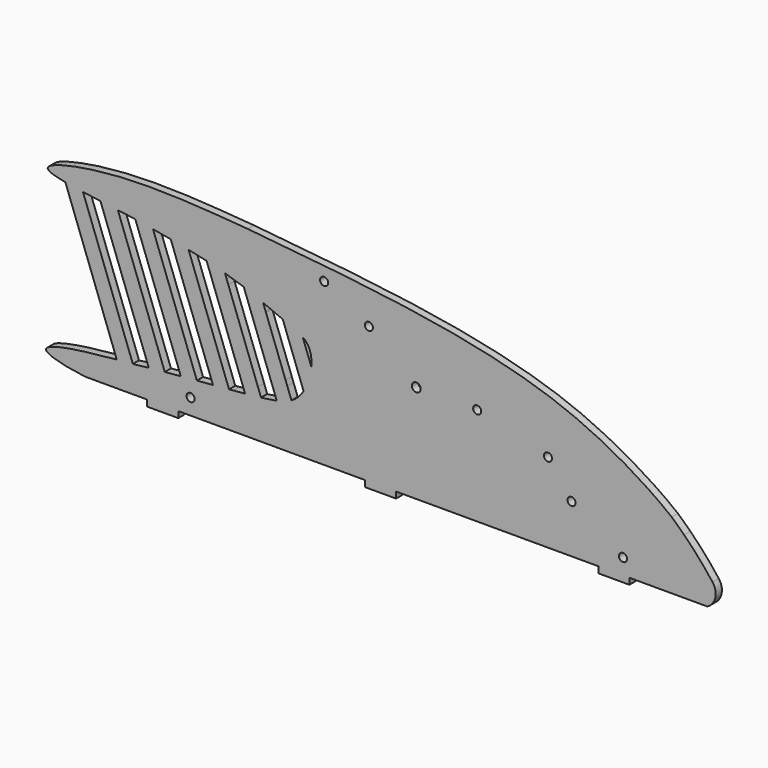
from build123d import *

# Parameters (mm, degrees)
F0_R     = 1.651
F0_R_2   = 1.8061142709
F1_DEPTH = 3.175


# Not quite as in the source:
# - a feature names something its author has since deleted; it is built from what else it names


with BuildPart() as f1:
    # F0 (on Front) → F1 (new body)
    with BuildSketch(Plane.XZ):
        with BuildLine():
            ThreePointArc((101.8242157669, -34.1397491809), (105.0796274749, -29.8955539863), (103.9375609563, -24.6699839404))
            ThreePointArc((103.9375609563, -24.6699839404), (98.381388832, -17.8735015058), (92.3581534987, -11.4872774041))
            ThreePointArc((92.3581534987, -11.4872774041), (89.8156936987, -9.0464347562), (87.2048720291, -6.6788569061))
            add(Edge.make_bspline(
                [(-85.6485664845, 40.5249372125), (-39.2165341594, 36.1134948801), (36.8475640649, 28.8975243931), (80.1105527935, -0.9081621475), (87.2048720291, -6.6788569061)],
                knots=[0, 0, 0, 0, 0.5343700027, 0.8750592741, 0.8750592741, 0.8750592741, 0.8750592741], degree=3))
            add(Edge.make_bspline(
                [(-166.859932426, 35.0105393748), (-167.0070818966, 35.1094314632), (-169.6480449533, 37.3313494106), (-138.9852615834, 44.7442194884), (-106.1222539211, 42.1445401212), (-85.6485664845, 40.5249372125)],
                knots=[0.4925129556, 0.4925129556, 0.4925129556, 0.4925129556, 0.5013804687, 0.6893595213, 1, 1, 1, 1], degree=3))
            add(Edge.make_bspline(
                [(-146.0141042884, 31.2589722541), (-151.9382775254, 32.1444047313), (-162.145842511, 33.6407441013), (-165.5296880535, 34.4446355916), (-166.859932426, 35.0105393748)],
                knots=[0.8656758918, 0.8656758918, 0.8656758918, 0.8656758918, 0.9278141873, 0.9914511144, 0.9914511144, 0.9914511144, 0.9914511144], degree=3))
            add(Edge.make_bspline(
                [(-133.5820238569, 29.35678448), (-137.9542479512, 30.0482442774), (-142.1697190197, 30.6843868334), (-146.0141042884, 31.2589722541)],
                knots=[0.8253523668, 0.8253523668, 0.8253523668, 0.8253523668, 0.8656758918, 0.8656758918, 0.8656758918, 0.8656758918], degree=3))
            add(Edge.make_bspline(
                [(-131.6806362519, 29.0942226068), (-132.3147563317, 29.1827732819), (-132.9488163176, 29.2702687124), (-133.5820238569, 29.35678448)],
                knots=[0.30311068, 0.30311068, 0.30311068, 0.30311068, 0.3105996727, 0.3105996727, 0.3105996727, 0.3105996727], degree=3))
            add(Edge.make_bspline(
                [(-124.5242243366, 28.0398482977), (-126.8819557506, 28.4091365836), (-129.2817260182, 28.759230659), (-131.6806362519, 29.0942226068)],
                knots=[0.2747794194, 0.2747794194, 0.2747794194, 0.2747794194, 0.30311068, 0.30311068, 0.30311068, 0.30311068], degree=3))
            add(Edge.make_bspline(
                [(-108.0116674089, 24.7705738209), (-112.7672708675, 26.0305747461), (-118.5089286797, 27.097680666), (-124.5242243366, 28.0398482977)],
                knots=[0.2024976878, 0.2024976878, 0.2024976878, 0.2024976878, 0.2747794194, 0.2747794194, 0.2747794194, 0.2747794194], degree=3))
            add(Edge.make_bspline(
                [(-102.5692031738, 23.558947235), (-104.3187177416, 23.9711384495), (-106.1393069255, 24.3752013047), (-108.0116674089, 24.7705738209)],
                knots=[0.7293104708, 0.7293104708, 0.7293104708, 0.7293104708, 0.7473852474, 0.7473852474, 0.7473852474, 0.7473852474], degree=3))
            add(Edge.make_bspline(
                [(-95.0830440369, 21.6100757598), (-96.2557735003, 21.9486690604), (-98.6537948613, 22.6077844658), (-101.252827931, 23.2488050276), (-102.5692031738, 23.558947235)],
                knots=[0.7016123961, 0.7016123961, 0.7016123961, 0.7016123961, 0.7157105906, 0.7293104708, 0.7293104708, 0.7293104708, 0.7293104708], degree=3))
            add(Edge.make_bspline(
                [(-87.404438233, 19.139158951), (-89.7270643692, 19.9661134917), (-92.2671026681, 20.7970503245), (-95.0830440369, 21.6100757598)],
                knots=[0.6677600115, 0.6677600115, 0.6677600115, 0.6677600115, 0.7016123961, 0.7016123961, 0.7016123961, 0.7016123961], degree=3))
            add(Edge.make_bspline(
                [(-79.5009681977, 16.0582584803), (-81.8655489773, 17.0490997411), (-84.4603298418, 18.0909300672), (-87.404438233, 19.139158951)],
                knots=[0.6248494938, 0.6248494938, 0.6248494938, 0.6248494938, 0.6677600115, 0.6677600115, 0.6677600115, 0.6677600115], degree=3))
            add(Edge.make_bspline(
                [(-71.4843313159, 12.6703730925), (-73.9521121546, 13.6621239816), (-76.5468977698, 14.8204006358), (-79.5009681977, 16.0582584803)],
                knots=[0.5712413903, 0.5712413903, 0.5712413903, 0.5712413903, 0.6248494938, 0.6248494938, 0.6248494938, 0.6248494938], degree=3))
            add(Edge.make_bspline(
                [(-63.3356655994, 8.9243363369), (-65.4352611539, 10.424736107), (-68.3578707481, 11.4139122272), (-71.4843313159, 12.6703730925)],
                knots=[0.5033246535, 0.5033246535, 0.5033246535, 0.5033246535, 0.5712413903, 0.5712413903, 0.5712413903, 0.5712413903], degree=3))
            add(Edge.make_bspline(
                [(-59.8424153153, -0.5517176671), (-59.5685681737, 2.4835120245), (-60.1606540756, 6.1658647467), (-62.6477224268, 8.4327227136), (-63.3356655994, 8.9243363369)],
                knots=[0.4110186684, 0.4110186684, 0.4110186684, 0.4110186684, 0.4810713889, 0.5033246535, 0.5033246535, 0.5033246535, 0.5033246535], degree=3))
            add(Edge.make_bspline(
                [(-63.0075179076, -10.3244698493), (-61.5384136321, -7.9164198493), (-60.3388409827, -4.449568462), (-59.8949280547, -1.1337512231), (-59.8424153153, -0.5517176671)],
                knots=[0.3356359982, 0.3356359982, 0.3356359982, 0.3356359982, 0.3975854069, 0.4110186684, 0.4110186684, 0.4110186684, 0.4110186684], degree=3))
            add(Edge.make_bspline(
                [(-67.9444449918, -15.2908373738), (-67.2102943656, -14.8703950623), (-65.3380336592, -13.5477151393), (-63.8223020979, -11.6600054557), (-63.0075179076, -10.3244698493)],
                knots=[0.2815826078, 0.2815826078, 0.2815826078, 0.2815826078, 0.3012780567, 0.3356359982, 0.3356359982, 0.3356359982, 0.3356359982], degree=3))
            add(Edge.make_bspline(
                [(-73.9382749374, -17.3901705387), (-71.6234415545, -16.908346885), (-69.6446238077, -16.2645164604), (-67.9444449918, -15.2908373738)],
                knots=[0.2359710075, 0.2359710075, 0.2359710075, 0.2359710075, 0.2815826078, 0.2815826078, 0.2815826078, 0.2815826078], degree=3))
            add(Edge.make_bspline(
                [(-80.3548864441, -18.3426345759), (-77.9680739947, -18.0724427195), (-75.8398049281, -17.785966683), (-73.9382749374, -17.3901705387)],
                knots=[0.1985031592, 0.1985031592, 0.1985031592, 0.1985031592, 0.2359710075, 0.2359710075, 0.2359710075, 0.2359710075], degree=3))
            add(Edge.make_bspline(
                [(-81.2421848416, -18.4411984354), (-80.9425135443, -18.4084739112), (-80.6467668076, -18.3756760061), (-80.3548864685, -18.3426345786)],
                knots=[0.1939212624, 0.1939212624, 0.1939212624, 0.1939212624, 0.1985031592, 0.1985031592, 0.1985031592, 0.1985031592], degree=3))
            add(Edge.make_bspline(
                [(-81.242184815, -18.4411984325), (-86.8235115185, -20.9425074888), (-91.5502384252, -21.2149262437), (-96.0113873436, -21.2686423497)],
                knots=[0.706684877, 0.706684877, 0.706684877, 0.706684877, 0.9497553414, 0.9497553414, 0.9497553414, 0.9497553414], degree=3))
            add(Edge.make_bspline(
                [(-96.0113873436, -21.2686423497), (-96.9335434145, -21.2797459094), (-97.8443517945, -21.2815046809), (-98.7490148928, -21.2916732166)],
                knots=[0.9497553414, 0.9497553414, 0.9497553414, 0.9497553414, 1, 1, 1, 1], degree=3))
            add(Edge.make_bspline(
                [(-133.305364874, -23.3117086185), (-122.8338263442, -22.475714872), (-110.8834436824, -21.7895004957), (-98.7490148928, -21.2916732166)],
                knots=[0.853722198, 0.853722198, 0.853722198, 0.853722198, 0.9841655102, 0.9841655102, 0.9841655102, 0.9841655102], degree=3))
            add(Edge.make_bspline(
                [(-139.2463766665, -23.8169718217), (-137.328523595, -23.6430585147), (-135.3449969617, -23.4745423478), (-133.305364874, -23.3117086185)],
                knots=[0.8283146263, 0.8283146263, 0.8283146263, 0.8283146263, 0.853722198, 0.853722198, 0.853722198, 0.853722198], degree=3))
            add(Edge.make_bspline(
                [(-152.2580874144, -34.1547166765), (-161.5981584725, -33.009893689), (-177.1137531043, -28.7902056183), (-155.6923384135, -25.3083121314), (-139.2463766665, -23.8169718217)],
                knots=[0.4265501578, 0.4265501578, 0.4265501578, 0.4265501578, 0.610439776, 0.8283146263, 0.8283146263, 0.8283146263, 0.8283146263], degree=3))
            ThreePointArc((-152.2580874144, -34.1547166765), (-152.2495450174, -34.155500254), (-152.2409707448, -34.1557617705))
            Line((-152.2409707448, -34.1557617705), (-126.8495585793, -34.1557617705))
            Line((-126.8495585793, -34.1557617705), (-126.8495585793, -35.5765540648))
            add(Edge.make_bspline(
                [(-114.1495585793, -35.5765321102), (-118.523301185, -35.6218647567), (-122.7687076518, -35.6265709825), (-126.8495585793, -35.5765540648)],
                knots=[0.2221019343, 0.2221019343, 0.2221019343, 0.2221019343, 0.2834552379, 0.2834552379, 0.2834552379, 0.2834552379], degree=3))
            Line((-114.1495585793, -35.5765321102), (-114.1495585793, -34.1557617705))
            Line((-114.1495585793, -34.1557617705), (-63.3228805236, -34.1557617705))
            Line((-63.3228805236, -34.1557617705), (-57.4806444347, -34.1557617705))
            Line((-57.4806444347, -34.1557617705), (-37.9495585793, -34.1557617705))
            Line((-37.9495585793, -34.1557617705), (-37.9495585793, -36.6983525455))
            Line((-37.9495585793, -36.6983525455), (-25.2495585793, -36.6983525455))
            Line((-25.2495585793, -36.6983525455), (-25.2495585793, -34.1583525455))
            Line((-25.2495585793, -34.1583525455), (-25.2495585793, -34.1557617705))
            Line((-25.2495585793, -34.1557617705), (57.3004414207, -34.1557617705))
            Line((57.3004414207, -34.1557617705), (57.3004414207, -36.6957617705))
            Line((57.3004414207, -36.6957617705), (70.0004414207, -36.6957617705))
            Line((70.0004414207, -36.6957617705), (70.0004414207, -34.1557617705))
            Line((70.0004414207, -34.1557617705), (101.7590292552, -34.1557617705))
            ThreePointArc((101.7590292552, -34.1557617705), (101.7925914524, -34.1516999913), (101.8242157669, -34.1397491809))
        make_face()
        with Locations((-109.1138124466, -27.6470873505)):
            Circle(F0_R, mode=Mode.SUBTRACT)
        with Locations((67.3906803131, -27.7224443853)):
            Circle(F0_R, mode=Mode.SUBTRACT)
        with Locations((46.3759977302, -14.4284265014)):
            Circle(F0_R, mode=Mode.SUBTRACT)
        with Locations((36.7670959526, -1.6008562954)):
            Circle(F0_R, mode=Mode.SUBTRACT)
        with Locations((-36.3425172139, 21.5731277197)):
            Circle(F0_R, mode=Mode.SUBTRACT)
        with Locations((-54.6054057777, 31.7963883281)):
            Circle(F0_R, mode=Mode.SUBTRACT)
        with Locations((-17.0012986666, 5.9441462856)):
            Circle(F0_R_2, mode=Mode.SUBTRACT)
        with Locations((7.8653013334, 5.9441462856)):
            Circle(F0_R, mode=Mode.SUBTRACT)
        with BuildLine():
            add(Edge.make_bspline(
                [(-146.0141042884, 31.2589722541), (-151.9382775254, 32.1444047313), (-162.145842511, 33.6407441013), (-165.5296880535, 34.4446355916), (-166.859932426, 35.0105393748)],
                knots=[0.8656758918, 0.8656758918, 0.8656758918, 0.8656758918, 0.9278141873, 0.9914511144, 0.9914511144, 0.9914511144, 0.9914511144], degree=3))
            add(Edge.make_bspline(
                [(-160.2262755413, 33.0946831043), (-163.4901021945, 33.703641199), (-165.8451335745, 34.3285418292), (-166.859932426, 35.0105393748)],
                knots=[0.4313592041, 0.4313592041, 0.4313592041, 0.4313592041, 0.4925129556, 0.4925129556, 0.4925129556, 0.4925129556], degree=3))
            add(Edge.make_bspline(
                [(-153.0349213305, 31.9455216907), (-155.7238859248, 32.329156746), (-158.1576206982, 32.7087177189), (-160.2262755413, 33.0946831043)],
                knots=[0.3925991786, 0.3925991786, 0.3925991786, 0.3925991786, 0.4313592041, 0.4313592041, 0.4313592041, 0.4313592041], degree=3))
            add(Edge.make_bspline(
                [(-145.911513117, 30.9806757105), (-148.4188378285, 31.3090067169), (-150.8139400572, 31.6286538986), (-153.0349213305, 31.9455216907)],
                knots=[0.3605848892, 0.3605848892, 0.3605848892, 0.3605848892, 0.3925991786, 0.3925991786, 0.3925991786, 0.3925991786], degree=3))
            Line((-145.911513117, 30.9806757105), (-146.0141042884, 31.2589722541))
        make_face()
        with BuildLine():
            add(Edge.make_bspline(
                [(-133.5820238569, 29.35678448), (-137.9542479512, 30.0482442774), (-142.1697190197, 30.6843868334), (-146.0141042884, 31.2589722541)],
                knots=[0.8253523668, 0.8253523668, 0.8253523668, 0.8253523668, 0.8656758918, 0.8656758918, 0.8656758918, 0.8656758918], degree=3))
            Line((-146.0141042884, 31.2589722541), (-145.911513117, 30.9806757105))
            add(Edge.make_bspline(
                [(-138.8022091808, 30.0540900559), (-141.2342218587, 30.373212682), (-143.6197455711, 30.6805716428), (-145.911513117, 30.9806757105)],
                knots=[0.3313228996, 0.3313228996, 0.3313228996, 0.3313228996, 0.3605848892, 0.3605848892, 0.3605848892, 0.3605848892], degree=3))
            add(Edge.make_bspline(
                [(-133.5820238569, 29.35678448), (-135.3342092326, 29.5961872878), (-137.0798672845, 29.8280886563), (-138.8022091808, 30.0540900559)],
                knots=[0.3105996727, 0.3105996727, 0.3105996727, 0.3105996727, 0.3313228996, 0.3313228996, 0.3313228996, 0.3313228996], degree=3))
        make_face()
        with BuildLine():
            add(Edge.make_bspline(
                [(-153.0349213305, 31.9455216907), (-155.7238859248, 32.329156746), (-158.1576206982, 32.7087177189), (-160.2262755413, 33.0946831043)],
                knots=[0.3925991786, 0.3925991786, 0.3925991786, 0.3925991786, 0.4313592041, 0.4313592041, 0.4313592041, 0.4313592041], degree=3))
            Line((-160.2262755413, 33.0946831043), (-139.2463766665, -23.8169718217))
            add(Edge.make_bspline(
                [(-139.2463766665, -23.8169718217), (-137.328523595, -23.6430585147), (-135.3449969617, -23.4745423478), (-133.305364874, -23.3117086185)],
                knots=[0.8283146263, 0.8283146263, 0.8283146263, 0.8283146263, 0.853722198, 0.853722198, 0.853722198, 0.853722198], degree=3))
            add(Edge.make_bspline(
                [(-133.305364874, -23.3117086185), (-133.1004170164, -23.2884499459), (-132.895464166, -23.2652975185), (-132.6905143301, -23.2422500801)],
                knots=[0, 0, 0, 0, 0.0020208288, 0.0020208288, 0.0020208288, 0.0020208288], degree=3))
            Line((-132.6905143301, -23.2422500801), (-153.0349213305, 31.9455216907))
        make_face()
        with BuildLine():
            add(Edge.make_bspline(
                [(-131.6806362519, 29.0942226068), (-132.3147563317, 29.1827732819), (-132.9488163176, 29.2702687124), (-133.5820238569, 29.35678448)],
                knots=[0.30311068, 0.30311068, 0.30311068, 0.30311068, 0.3105996727, 0.3105996727, 0.3105996727, 0.3105996727], degree=3))
            add(Edge.make_bspline(
                [(-131.6649143971, 29.0515743188), (-132.3068274232, 29.1544685142), (-132.9460837508, 29.2562116349), (-133.5820238569, 29.35678448)],
                knots=[0.8194873091, 0.8194873091, 0.8194873091, 0.8194873091, 0.8253523668, 0.8253523668, 0.8253523668, 0.8253523668], degree=3))
            Line((-131.6649143971, 29.0515743188), (-131.6806362519, 29.0942226068))
        make_face()
        with BuildLine():
            add(Edge.make_bspline(
                [(-138.8022091808, 30.0540900559), (-141.2342218587, 30.373212682), (-143.6197455711, 30.6805716428), (-145.911513117, 30.9806757105)],
                knots=[0.3313228996, 0.3313228996, 0.3313228996, 0.3313228996, 0.3605848892, 0.3605848892, 0.3605848892, 0.3605848892], degree=3))
            Line((-145.911513117, 30.9806757105), (-126.2084949262, -22.4672164347))
            Line((-126.2084949262, -22.4672164347), (-126.1805877741, -22.5429194788))
            add(Edge.make_bspline(
                [(-126.1805877741, -22.5429194788), (-123.9904993464, -22.3178624533), (-121.8105472714, -22.1033724676), (-119.6506417586, -21.8978951719)],
                knots=[0.0234517677, 0.0234517677, 0.0234517677, 0.0234517677, 0.0451483955, 0.0451483955, 0.0451483955, 0.0451483955], degree=3))
            Line((-119.6506417586, -21.8978951719), (-138.8022091808, 30.0540900559))
        make_face()
        with BuildLine():
            Line((-131.6806362519, 29.0942226068), (-131.6649143971, 29.0515743188))
            add(Edge.make_bspline(
                [(-124.4587574049, 27.8622577646), (-126.8749129775, 28.2738277576), (-129.2881250019, 28.6705915024), (-131.6649143971, 29.0515743188)],
                knots=[0.7977709605, 0.7977709605, 0.7977709605, 0.7977709605, 0.8194873091, 0.8194873091, 0.8194873091, 0.8194873091], degree=3))
            Line((-124.4587574049, 27.8622577646), (-124.5242243366, 28.0398482977))
            add(Edge.make_bspline(
                [(-124.5242243366, 28.0398482977), (-126.8819557506, 28.4091365836), (-129.2817260182, 28.759230659), (-131.6806362519, 29.0942226068)],
                knots=[0.2747794194, 0.2747794194, 0.2747794194, 0.2747794194, 0.30311068, 0.30311068, 0.30311068, 0.30311068], degree=3))
        make_face()
        with BuildLine():
            add(Edge.make_bspline(
                [(-124.4587574049, 27.8622577646), (-126.8749129775, 28.2738277576), (-129.2881250019, 28.6705915024), (-131.6649143971, 29.0515743188)],
                knots=[0.7977709605, 0.7977709605, 0.7977709605, 0.7977709605, 0.8194873091, 0.8194873091, 0.8194873091, 0.8194873091], degree=3))
            Line((-131.6649143971, 29.0515743188), (-113.1052410481, -21.2947944356))
            add(Edge.make_bspline(
                [(-113.1052410481, -21.2947944356), (-110.8824432445, -21.0958896664), (-108.6931707163, -20.9052358248), (-106.5490323993, -20.7210121272)],
                knots=[0.0673104273, 0.0673104273, 0.0673104273, 0.0673104273, 0.0901819686, 0.0901819686, 0.0901819686, 0.0901819686], degree=3))
            Line((-106.5490323993, -20.7210121272), (-124.4587574049, 27.8622577646))
        make_face()
        with BuildLine():
            add(Edge.make_bspline(
                [(-132.6905143301, -23.2422500801), (-130.5170162436, -22.9978314259), (-128.3438571985, -22.7652205402), (-126.1805877741, -22.5429194788)],
                knots=[0.0020208288, 0.0020208288, 0.0020208288, 0.0020208288, 0.0234517677, 0.0234517677, 0.0234517677, 0.0234517677], degree=3))
            add(Edge.make_bspline(
                [(-133.305364874, -23.3117086185), (-133.1004170164, -23.2884499459), (-132.895464166, -23.2652975185), (-132.6905143301, -23.2422500801)],
                knots=[0, 0, 0, 0, 0.0020208288, 0.0020208288, 0.0020208288, 0.0020208288], degree=3))
            add(Edge.make_bspline(
                [(-133.305364874, -23.3117086185), (-122.8338263442, -22.475714872), (-110.8834436824, -21.7895004957), (-98.7490148928, -21.2916732166)],
                knots=[0.853722198, 0.853722198, 0.853722198, 0.853722198, 0.9841655102, 0.9841655102, 0.9841655102, 0.9841655102], degree=3))
            add(Edge.make_bspline(
                [(-98.7490148928, -21.2916732166), (-97.7639622967, -21.2512604323), (-96.7776968514, -21.2120891039), (-95.7909112202, -21.174179885)],
                knots=[0.9841655102, 0.9841655102, 0.9841655102, 0.9841655102, 0.9947546797, 0.9947546797, 0.9947546797, 0.9947546797], degree=3))
            add(Edge.make_bspline(
                [(-91.8007028901, -19.4584197408), (-93.1232258666, -20.0303526691), (-94.4561565841, -20.6022678336), (-95.7909112202, -21.174179885)],
                knots=[0.9537015671, 0.9537015671, 0.9537015671, 0.9537015671, 0.9918863691, 0.9918863691, 0.9918863691, 0.9918863691], degree=3))
            add(Edge.make_bspline(
                [(-93.4265039677, -19.6008757346), (-92.8786151945, -19.5531958217), (-92.336588061, -19.5057251461), (-91.8007028901, -19.4584197408)],
                knots=[0.1394929365, 0.1394929365, 0.1394929365, 0.1394929365, 0.1461036875, 0.1461036875, 0.1461036875, 0.1461036875], degree=3))
            add(Edge.make_bspline(
                [(-99.987241926, -20.1623714966), (-97.7243605002, -19.9704519625), (-95.5321437404, -19.784118622), (-93.4265039677, -19.6008757346)],
                knots=[0.1140865752, 0.1140865752, 0.1140865752, 0.1140865752, 0.1394929365, 0.1394929365, 0.1394929365, 0.1394929365], degree=3))
            add(Edge.make_bspline(
                [(-106.5490323993, -20.7210121272), (-104.3080473179, -20.5284673856), (-102.1163657866, -20.342946782), (-99.987241926, -20.1623714966)],
                knots=[0.0901819686, 0.0901819686, 0.0901819686, 0.0901819686, 0.1140865752, 0.1140865752, 0.1140865752, 0.1140865752], degree=3))
            add(Edge.make_bspline(
                [(-113.1052410481, -21.2947944356), (-110.8824432445, -21.0958896664), (-108.6931707163, -20.9052358248), (-106.5490323993, -20.7210121272)],
                knots=[0.0673104273, 0.0673104273, 0.0673104273, 0.0673104273, 0.0901819686, 0.0901819686, 0.0901819686, 0.0901819686], degree=3))
            add(Edge.make_bspline(
                [(-119.6506417586, -21.8978951719), (-117.4444051423, -21.6880102808), (-115.2590843306, -21.4875288805), (-113.1052410481, -21.2947944356)],
                knots=[0.0451483955, 0.0451483955, 0.0451483955, 0.0451483955, 0.0673104273, 0.0673104273, 0.0673104273, 0.0673104273], degree=3))
            add(Edge.make_bspline(
                [(-126.1805877741, -22.5429194788), (-123.9904993464, -22.3178624533), (-121.8105472714, -22.1033724676), (-119.6506417586, -21.8978951719)],
                knots=[0.0234517677, 0.0234517677, 0.0234517677, 0.0234517677, 0.0451483955, 0.0451483955, 0.0451483955, 0.0451483955], degree=3))
        make_face()
        with BuildLine():
            Line((-124.5242243366, 28.0398482977), (-124.4587574049, 27.8622577646))
            add(Edge.make_bspline(
                [(-117.2187514903, 26.5811200726), (-119.6125726628, 27.0223849911), (-122.0371434652, 27.4497579888), (-124.4587574049, 27.8622577646)],
                knots=[0.7760055522, 0.7760055522, 0.7760055522, 0.7760055522, 0.7977709605, 0.7977709605, 0.7977709605, 0.7977709605], degree=3))
            add(Edge.make_bspline(
                [(-109.9305159939, 25.1691511818), (-112.3022395164, 25.6539310572), (-114.7440643866, 26.1249487363), (-117.2187514903, 26.5811200726)],
                knots=[0.7535048843, 0.7535048843, 0.7535048843, 0.7535048843, 0.7760055522, 0.7760055522, 0.7760055522, 0.7760055522], degree=3))
            add(Edge.make_bspline(
                [(-108.0116674089, 24.7705738209), (-108.6455986912, 24.9044364015), (-109.2854646151, 25.0373027922), (-109.9305159939, 25.1691511818)],
                knots=[0.7473852474, 0.7473852474, 0.7473852474, 0.7473852474, 0.7535048843, 0.7535048843, 0.7535048843, 0.7535048843], degree=3))
            add(Edge.make_bspline(
                [(-108.0116674089, 24.7705738209), (-112.7672708675, 26.0305747461), (-118.5089286797, 27.097680666), (-124.5242243366, 28.0398482977)],
                knots=[0.2024976878, 0.2024976878, 0.2024976878, 0.2024976878, 0.2747794194, 0.2747794194, 0.2747794194, 0.2747794194], degree=3))
        make_face()
        with BuildLine():
            add(Edge.make_bspline(
                [(-114.1495585793, -35.5765321102), (-118.523301185, -35.6218647567), (-122.7687076518, -35.6265709825), (-126.8495585793, -35.5765540648)],
                knots=[0.2221019343, 0.2221019343, 0.2221019343, 0.2221019343, 0.2834552379, 0.2834552379, 0.2834552379, 0.2834552379], degree=3))
            Line((-126.8495585793, -35.5765540648), (-126.8495585793, -36.6957617705))
            Line((-126.8495585793, -36.6957617705), (-114.1495585793, -36.6957617705))
            Line((-114.1495585793, -36.6957617705), (-114.1495585793, -35.5765321102))
        make_face()
        with BuildLine():
            add(Edge.make_bspline(
                [(-98.7490148928, -21.2916732166), (-97.7639622967, -21.2512604323), (-96.7776968514, -21.2120891039), (-95.7909112202, -21.174179885)],
                knots=[0.9841655102, 0.9841655102, 0.9841655102, 0.9841655102, 0.9947546797, 0.9947546797, 0.9947546797, 0.9947546797], degree=3))
            add(Edge.make_bspline(
                [(-96.0113873436, -21.2686423497), (-96.9335434145, -21.2797459094), (-97.8443517945, -21.2815046809), (-98.7490148928, -21.2916732166)],
                knots=[0.9497553414, 0.9497553414, 0.9497553414, 0.9497553414, 1, 1, 1, 1], degree=3))
            add(Edge.make_bspline(
                [(-95.7909112202, -21.174179885), (-95.8643982082, -21.2056673906), (-95.9378907249, -21.2371548868), (-96.0113873378, -21.268642376)],
                knots=[0.9918863691, 0.9918863691, 0.9918863691, 0.9918863691, 0.9939886926, 0.9939886926, 0.9939886926, 0.9939886926], degree=3))
        make_face()
        with BuildLine():
            add(Edge.make_bspline(
                [(-109.9305159939, 25.1691511818), (-112.3022395164, 25.6539310572), (-114.7440643866, 26.1249487363), (-117.2187514903, 26.5811200726)],
                knots=[0.7535048843, 0.7535048843, 0.7535048843, 0.7535048843, 0.7760055522, 0.7760055522, 0.7760055522, 0.7760055522], degree=3))
            Line((-117.2187514903, 26.5811200726), (-99.987241926, -20.1623714966))
            add(Edge.make_bspline(
                [(-99.987241926, -20.1623714966), (-97.7243605002, -19.9704519625), (-95.5321437404, -19.784118622), (-93.4265039677, -19.6008757346)],
                knots=[0.1140865752, 0.1140865752, 0.1140865752, 0.1140865752, 0.1394929365, 0.1394929365, 0.1394929365, 0.1394929365], degree=3))
            Line((-93.4265039677, -19.6008757346), (-109.9305159939, 25.1691511818))
        make_face()
        with BuildLine():
            add(Edge.make_bspline(
                [(-91.8007028901, -19.4584197408), (-93.1232258666, -20.0303526691), (-94.4561565841, -20.6022678336), (-95.7909112202, -21.174179885)],
                knots=[0.9537015671, 0.9537015671, 0.9537015671, 0.9537015671, 0.9918863691, 0.9918863691, 0.9918863691, 0.9918863691], degree=3))
            add(Edge.make_bspline(
                [(-95.7909112202, -21.174179885), (-95.8643982082, -21.2056673906), (-95.9378907249, -21.2371548868), (-96.0113873378, -21.268642376)],
                knots=[0.9918863691, 0.9918863691, 0.9918863691, 0.9918863691, 0.9939886926, 0.9939886926, 0.9939886926, 0.9939886926], degree=3))
            add(Edge.make_bspline(
                [(-81.242184815, -18.4411984325), (-86.8235115185, -20.9425074888), (-91.5502384252, -21.2149262437), (-96.0113873436, -21.2686423497)],
                knots=[0.706684877, 0.706684877, 0.706684877, 0.706684877, 0.9497553414, 0.9497553414, 0.9497553414, 0.9497553414], degree=3))
            add(Edge.make_bspline(
                [(-86.8765772789, -19.0100525082), (-84.8769444797, -18.8209932024), (-82.9926132911, -18.6323476668), (-81.2421848416, -18.4411984354)],
                knots=[0.1671576631, 0.1671576631, 0.1671576631, 0.1671576631, 0.1939212624, 0.1939212624, 0.1939212624, 0.1939212624], degree=3))
            add(Edge.make_bspline(
                [(-91.8007028901, -19.4584197408), (-90.0940112569, -19.3077610852), (-88.4496175808, -19.1587787681), (-86.8765772789, -19.0100525082)],
                knots=[0.1461036875, 0.1461036875, 0.1461036875, 0.1461036875, 0.1671576631, 0.1671576631, 0.1671576631, 0.1671576631], degree=3))
        make_face()
        with BuildLine():
            add(Edge.make_bspline(
                [(-95.0830440369, 21.6100757598), (-96.2557735003, 21.9486690604), (-98.6537948613, 22.6077844658), (-101.252827931, 23.2488050276), (-102.5692031738, 23.558947235)],
                knots=[0.7016123961, 0.7016123961, 0.7016123961, 0.7016123961, 0.7157105906, 0.7293104708, 0.7293104708, 0.7293104708, 0.7293104708], degree=3))
            Line((-102.5692031738, 23.558947235), (-102.3586580437, 22.9878066466))
            add(Edge.make_bspline(
                [(-100.3286994702, 22.1462184152), (-100.9667307172, 22.4336146948), (-101.6422894477, 22.7143386396), (-102.3586580437, 22.9878066466)],
                knots=[0.1569312578, 0.1569312578, 0.1569312578, 0.1569312578, 0.1706574214, 0.1706574214, 0.1706574214, 0.1706574214], degree=3))
            add(Edge.make_bspline(
                [(-100.3286994703, 22.1462184152), (-98.3419538443, 21.370808658), (-96.3670610524, 20.5954191311), (-94.4231813629, 19.820082537)],
                knots=[0.0317602035, 0.0317602035, 0.0317602035, 0.0317602035, 0.0831010058, 0.0831010058, 0.0831010058, 0.0831010058], degree=3))
            Line((-94.4231813629, 19.820082537), (-95.0830440369, 21.6100757598))
        make_face()
        with BuildLine():
            add(Edge.make_bspline(
                [(-86.8765772789, -19.0100525082), (-84.8769444797, -18.8209932024), (-82.9926132911, -18.6323476668), (-81.2421848416, -18.4411984354)],
                knots=[0.1671576631, 0.1671576631, 0.1671576631, 0.1671576631, 0.1939212624, 0.1939212624, 0.1939212624, 0.1939212624], degree=3))
            add(Edge.make_bspline(
                [(-80.4533326205, -18.075582058), (-80.7178914258, -18.2021897286), (-80.9809740433, -18.3241350704), (-81.242184815, -18.4411984325)],
                knots=[0.6953089753, 0.6953089753, 0.6953089753, 0.6953089753, 0.706684877, 0.706684877, 0.706684877, 0.706684877], degree=3))
            Line((-80.4533326205, -18.075582058), (-81.6267561876, -14.89246485))
            add(Edge.make_bspline(
                [(-81.6267561876, -14.89246485), (-83.488541827, -15.7754334505), (-85.4295143068, -16.6582668958), (-87.418121426, -17.5410190391)],
                knots=[0.8521015775, 0.8521015775, 0.8521015775, 0.8521015775, 0.9110320857, 0.9110320857, 0.9110320857, 0.9110320857], degree=3))
            Line((-87.4181214259, -17.5410190391), (-86.8765772789, -19.0100525082))
        make_face()
        with BuildLine():
            add(Edge.make_bspline(
                [(-80.4533326205, -18.075582058), (-80.7178914258, -18.2021897286), (-80.9809740433, -18.3241350704), (-81.242184815, -18.4411984325)],
                knots=[0.6953089753, 0.6953089753, 0.6953089753, 0.6953089753, 0.706684877, 0.706684877, 0.706684877, 0.706684877], degree=3))
            add(Edge.make_bspline(
                [(-81.2421848416, -18.4411984354), (-80.9425135443, -18.4084739112), (-80.6467668076, -18.3756760061), (-80.3548864685, -18.3426345786)],
                knots=[0.1939212624, 0.1939212624, 0.1939212624, 0.1939212624, 0.1985031592, 0.1985031592, 0.1985031592, 0.1985031592], degree=3))
            Line((-80.3548864441, -18.3426345759), (-80.4533326205, -18.075582058))
        make_face()
        with BuildLine():
            add(Edge.make_bspline(
                [(-100.3286994702, 22.1462184152), (-100.9667307172, 22.4336146948), (-101.6422894477, 22.7143386396), (-102.3586580437, 22.9878066466)],
                knots=[0.1569312578, 0.1569312578, 0.1569312578, 0.1569312578, 0.1706574214, 0.1706574214, 0.1706574214, 0.1706574214], degree=3))
            Line((-102.3586580437, 22.9878066466), (-102.3368731501, 22.9287113022))
            add(Edge.make_bspline(
                [(-102.3368731501, 22.9287113022), (-101.6666269569, 22.6678788806), (-100.9969926472, 22.4070475034), (-100.3286994703, 22.1462184152)],
                knots=[0.0144903994, 0.0144903994, 0.0144903994, 0.0144903994, 0.0317602035, 0.0317602035, 0.0317602035, 0.0317602035], degree=3))
        make_face()
        with BuildLine():
            add(Edge.make_bspline(
                [(-102.3368731501, 22.9287113022), (-101.6666269569, 22.6678788806), (-100.9969926472, 22.4070475034), (-100.3286994703, 22.1462184152)],
                knots=[0.0144903994, 0.0144903994, 0.0144903994, 0.0144903994, 0.0317602035, 0.0317602035, 0.0317602035, 0.0317602035], degree=3))
            Line((-102.3368731501, 22.9287113022), (-87.4181214259, -17.5410190391))
            add(Edge.make_bspline(
                [(-81.6267561876, -14.89246485), (-83.488541827, -15.7754334505), (-85.4295143068, -16.6582668958), (-87.418121426, -17.5410190391)],
                knots=[0.8521015775, 0.8521015775, 0.8521015775, 0.8521015775, 0.9110320857, 0.9110320857, 0.9110320857, 0.9110320857], degree=3))
            Line((-81.6267561876, -14.89246485), (-93.7330933839, 17.9480978737))
            add(Edge.make_bspline(
                [(-93.7330933839, 17.9480978737), (-95.3779897097, 19.4459076442), (-97.4790442928, 20.862613106), (-100.3286994702, 22.1462184152)],
                knots=[0.0956257444, 0.0956257444, 0.0956257444, 0.0956257444, 0.1569312578, 0.1569312578, 0.1569312578, 0.1569312578], degree=3))
        make_face()
        with BuildLine():
            add(Edge.make_bspline(
                [(-79.5009681977, 16.0582584803), (-81.8655489773, 17.0490997411), (-84.4603298418, 18.0909300672), (-87.404438233, 19.139158951)],
                knots=[0.6248494938, 0.6248494938, 0.6248494938, 0.6248494938, 0.6677600115, 0.6677600115, 0.6677600115, 0.6677600115], degree=3))
            Line((-87.404438233, 19.139158951), (-86.4479529651, 16.5445249237))
            add(Edge.make_bspline(
                [(-86.4479529651, 16.5445249237), (-83.569113096, 15.317450314), (-80.8356242299, 14.0906237876), (-78.3235020587, 12.8641750869)],
                knots=[0.1554096519, 0.1554096519, 0.1554096519, 0.1554096519, 0.2366858177, 0.2366858177, 0.2366858177, 0.2366858177], degree=3))
            Line((-78.3235020587, 12.8641750869), (-78.4705088009, 13.2629566556))
            Line((-78.4705088009, 13.2629566556), (-79.5009681977, 16.0582584803))
        make_face()
        with BuildLine():
            Line((-93.7330933839, 17.9480978737), (-94.4231813629, 19.820082537))
            add(Edge.make_bspline(
                [(-100.3286994703, 22.1462184152), (-98.3419538443, 21.370808658), (-96.3670610524, 20.5954191311), (-94.4231813629, 19.820082537)],
                knots=[0.0317602035, 0.0317602035, 0.0317602035, 0.0317602035, 0.0831010058, 0.0831010058, 0.0831010058, 0.0831010058], degree=3))
            add(Edge.make_bspline(
                [(-93.7330933839, 17.9480978737), (-95.3779897097, 19.4459076442), (-97.4790442928, 20.862613106), (-100.3286994702, 22.1462184152)],
                knots=[0.0956257444, 0.0956257444, 0.0956257444, 0.0956257444, 0.1569312578, 0.1569312578, 0.1569312578, 0.1569312578], degree=3))
        make_face()
        with BuildLine():
            Line((-75.9134393546, -12.032190674), (-74.8757131773, -14.8472049149))
            add(Edge.make_bspline(
                [(-69.6391231548, -10.6937256625), (-71.2345751528, -12.1809764556), (-73.0245429706, -13.590139347), (-74.8757131773, -14.8472049149)],
                knots=[0.5373650724, 0.5373650724, 0.5373650724, 0.5373650724, 0.616524715, 0.616524715, 0.616524715, 0.616524715], degree=3))
            Line((-69.6391231548, -10.6937256625), (-70.3545693652, -8.7529523495))
            add(Edge.make_bspline(
                [(-70.3545693652, -8.7529523495), (-71.9943852255, -9.846395577), (-73.8672537346, -10.9394410332), (-75.9134393546, -12.032190674)],
                knots=[0.7155784548, 0.7155784548, 0.7155784548, 0.7155784548, 0.788480754, 0.788480754, 0.788480754, 0.788480754], degree=3))
        make_face()
        with BuildLine():
            add(Edge.make_bspline(
                [(-69.6391231548, -10.6937256625), (-71.2345751528, -12.1809764556), (-73.0245429706, -13.590139347), (-74.8757131773, -14.8472049149)],
                knots=[0.5373650724, 0.5373650724, 0.5373650724, 0.5373650724, 0.616524715, 0.616524715, 0.616524715, 0.616524715], degree=3))
            Line((-74.8757131773, -14.8472049149), (-73.9382749374, -17.3901705387))
            add(Edge.make_bspline(
                [(-73.9382749374, -17.3901705387), (-71.6234415545, -16.908346885), (-69.6446238077, -16.2645164604), (-67.9444449918, -15.2908373738)],
                knots=[0.2359710075, 0.2359710075, 0.2359710075, 0.2359710075, 0.2815826078, 0.2815826078, 0.2815826078, 0.2815826078], degree=3))
            Line((-67.9444449918, -15.2908373738), (-69.6391231548, -10.6937256625))
        make_face()
        with BuildLine():
            add(Edge.make_bspline(
                [(-86.4479529651, 16.5445249237), (-83.569113096, 15.317450314), (-80.8356242299, 14.0906237876), (-78.3235020587, 12.8641750869)],
                knots=[0.1554096519, 0.1554096519, 0.1554096519, 0.1554096519, 0.2366858177, 0.2366858177, 0.2366858177, 0.2366858177], degree=3))
            Line((-86.4479529651, 16.5445249237), (-75.9134393546, -12.032190674))
            add(Edge.make_bspline(
                [(-70.3545693652, -8.7529523495), (-71.9943852255, -9.846395577), (-73.8672537346, -10.9394410332), (-75.9134393546, -12.032190674)],
                knots=[0.7155784548, 0.7155784548, 0.7155784548, 0.7155784548, 0.788480754, 0.788480754, 0.788480754, 0.788480754], degree=3))
            Line((-70.3545693652, -8.7529523495), (-78.3235020587, 12.8641750869))
        make_face()
        with BuildLine():
            add(Edge.make_bspline(
                [(-63.3356655994, 8.9243363369), (-65.4352611539, 10.424736107), (-68.3578707481, 11.4139122272), (-71.4843313159, 12.6703730925)],
                knots=[0.5033246535, 0.5033246535, 0.5033246535, 0.5033246535, 0.5712413903, 0.5712413903, 0.5712413903, 0.5712413903], degree=3))
            Line((-71.4843313159, 12.6703730925), (-70.0216425392, 8.7025732753))
            add(Edge.make_bspline(
                [(-70.0216425392, 8.7025732753), (-66.0716713944, 6.1218356889), (-63.3996109488, 3.3038450992), (-63.3404701948, 0)],
                knots=[0.1733665209, 0.1733665209, 0.1733665209, 0.1733665209, 0.3536105588, 0.3536105588, 0.3536105588, 0.3536105588], degree=3))
            add(Edge.make_bspline(
                [(-63.3404701953, 1.86e-08), (-63.3386710798, -0.0738103901), (-63.3386500644, -0.1476177639), (-63.3403889178, -0.2214221341)],
                knots=[0.5212834356, 0.5212834356, 0.5212834356, 0.5212834356, 0.5261917719, 0.5261917719, 0.5261917719, 0.5261917719], degree=3))
            add(Edge.make_bspline(
                [(-63.340388918, -0.2214221524), (-63.3666903447, -1.77071701), (-63.9526638994, -3.4212699454), (-64.9391059632, -5.0846985075)],
                knots=[0.3576242145, 0.3576242145, 0.3576242145, 0.3576242145, 0.4416082686, 0.4416082686, 0.4416082686, 0.4416082686], degree=3))
            Line((-64.9391059632, -5.0846985075), (-63.0075179076, -10.3244698493))
            add(Edge.make_bspline(
                [(-63.0075179076, -10.3244698493), (-61.5384136321, -7.9164198493), (-60.3388409827, -4.449568462), (-59.8949280547, -1.1337512231), (-59.8424153153, -0.5517176671)],
                knots=[0.3356359982, 0.3356359982, 0.3356359982, 0.3356359982, 0.3975854069, 0.4110186684, 0.4110186684, 0.4110186684, 0.4110186684], degree=3))
            Line((-59.8424153153, -0.5517176671), (-63.3356655994, 8.9243363369))
        make_face()
        with BuildLine():
            Line((-65.1938680372, -4.3936117045), (-64.9391059632, -5.0846985075))
            add(Edge.make_bspline(
                [(-63.340388918, -0.2214221524), (-63.3666903447, -1.77071701), (-63.9526638994, -3.4212699454), (-64.9391059632, -5.0846985075)],
                knots=[0.3576242145, 0.3576242145, 0.3576242145, 0.3576242145, 0.4416082686, 0.4416082686, 0.4416082686, 0.4416082686], degree=3))
            add(Edge.make_bspline(
                [(-63.340388918, -0.2214221524), (-63.3731784674, -1.6131505364), (-64.0317530006, -3.0038108387), (-65.1938680372, -4.3936117045)],
                knots=[0.5261917719, 0.5261917719, 0.5261917719, 0.5261917719, 0.6187482284, 0.6187482284, 0.6187482284, 0.6187482284], degree=3))
        make_face()
        with BuildLine():
            add(Edge.make_bspline(
                [(-70.0216425392, 8.7025732753), (-66.0716713944, 6.1218356889), (-63.3996109488, 3.3038450992), (-63.3404701948, 0)],
                knots=[0.1733665209, 0.1733665209, 0.1733665209, 0.1733665209, 0.3536105588, 0.3536105588, 0.3536105588, 0.3536105588], degree=3))
            Line((-70.0216425392, 8.7025732753), (-69.7859129424, 8.0631154041))
            add(Edge.make_bspline(
                [(-69.7859129424, 8.0631154041), (-65.8227645505, 5.3723130184), (-63.4058958645, 2.6841498122), (-63.3404701953, 1.86e-08)],
                knots=[0.3427895049, 0.3427895049, 0.3427895049, 0.3427895049, 0.5212834356, 0.5212834356, 0.5212834356, 0.5212834356], degree=3))
        make_face()
        with BuildLine():
            add(Edge.make_bspline(
                [(-69.7859129424, 8.0631154041), (-65.8227645505, 5.3723130184), (-63.4058958645, 2.6841498122), (-63.3404701953, 1.86e-08)],
                knots=[0.3427895049, 0.3427895049, 0.3427895049, 0.3427895049, 0.5212834356, 0.5212834356, 0.5212834356, 0.5212834356], degree=3))
            Line((-69.7859129424, 8.0631154041), (-65.1938680372, -4.3936117045))
            add(Edge.make_bspline(
                [(-63.340388918, -0.2214221524), (-63.3731784674, -1.6131505364), (-64.0317530006, -3.0038108387), (-65.1938680372, -4.3936117045)],
                knots=[0.5261917719, 0.5261917719, 0.5261917719, 0.5261917719, 0.6187482284, 0.6187482284, 0.6187482284, 0.6187482284], degree=3))
            add(Edge.make_bspline(
                [(-63.3404701948, 0), (-63.3391532546, -0.0735696844), (-63.3391319547, -0.1473802842), (-63.340388918, -0.2214221524)],
                knots=[0.3536105588, 0.3536105588, 0.3536105588, 0.3536105588, 0.3576242145, 0.3576242145, 0.3576242145, 0.3576242145], degree=3))
        make_face()
    extrude(amount=F1_DEPTH)


solid = f1.part
